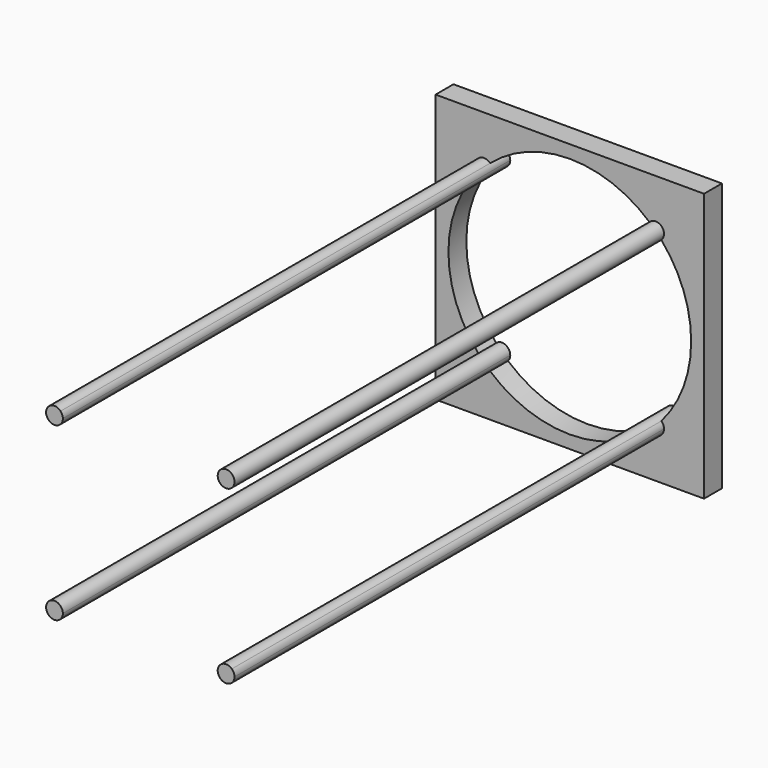
from build123d import *

# Parameters (mm, degrees)
F1_DEPTH = 635
F0_W     = 304.8
F0_H     = 304.8
F2_DEPTH = 25.4


with BuildPart() as f1:
    # F0 (on Front) → F1 (new body)
    with BuildSketch(Plane.XZ):
        with BuildLine():
            ThreePointArc((79.0087948248, 92.4711311021), (79.2375540094, 79.2375540094), (92.4711311021, 79.0087948248))
            ThreePointArc((92.4711311021, 79.0087948248), (85.9727461002, 85.9727461002), (79.0087948248, 92.4711311021))
        make_face()
        with BuildLine():
            ThreePointArc((79.0087948248, 92.4711311021), (85.9727461002, 85.9727461002), (92.4711311021, 79.0087948248))
            ThreePointArc((92.4711311021, 79.0087948248), (94.708384089, 82.1761352526), (95.4977461002, 85.9727461002))
            ThreePointArc((95.4977461002, 85.9727461002), (89.4651656842, 94.834384236), (79.0087948248, 92.4711311021))
        make_face()
    extrude(amount=F1_DEPTH)


with BuildPart() as f1b:
    # F0 (on Front) → F1, piece 2 (new body)
    with BuildSketch(Plane.XZ):
        with BuildLine():
            ThreePointArc((95.4977461002, -108.898811727), (94.708384089, -105.1022008793), (92.4711311021, -101.9348604515))
            ThreePointArc((92.4711311021, -101.9348604515), (85.9727461002, -108.898811727), (79.0087948248, -115.3971967289))
            ThreePointArc((79.0087948248, -115.3971967289), (89.4651656842, -117.7604498627), (95.4977461002, -108.898811727))
        make_face()
        with BuildLine():
            ThreePointArc((79.0087948248, -115.3971967289), (85.9727461002, -108.898811727), (92.4711311021, -101.9348604515))
            ThreePointArc((92.4711311021, -101.9348604515), (79.2375540094, -102.1636196362), (79.0087948248, -115.3971967289))
        make_face()
    extrude(amount=F1_DEPTH)


with BuildPart() as f1c:
    # F0 (on Front) → F1, piece 3 (new body)
    with BuildSketch(Plane.XZ):
        with BuildLine():
            ThreePointArc((-99.373811727, 85.9727461002), (-100.0371735912, 89.4651656842), (-101.9348604515, 92.4711311021))
            ThreePointArc((-101.9348604515, 92.4711311021), (-108.898811727, 85.9727461002), (-115.3971967289, 79.0087948248))
            ThreePointArc((-115.3971967289, 79.0087948248), (-105.1022008793, 77.2371081114), (-99.373811727, 85.9727461002))
        make_face()
        with BuildLine():
            ThreePointArc((-115.3971967289, 79.0087948248), (-108.898811727, 85.9727461002), (-101.9348604515, 92.4711311021))
            ThreePointArc((-101.9348604515, 92.4711311021), (-115.6340038178, 92.707938191), (-115.3971967289, 79.0087948248))
        make_face()
    extrude(amount=F1_DEPTH)


with BuildPart() as f1d:
    # F0 (on Front) → F1, piece 4 (new body)
    with BuildSketch(Plane.XZ):
        with BuildLine():
            ThreePointArc((-115.3971967289, -101.9348604515), (-115.6340038178, -115.6340038178), (-101.9348604515, -115.3971967289))
            ThreePointArc((-101.9348604515, -115.3971967289), (-108.898811727, -108.898811727), (-115.3971967289, -101.9348604515))
        make_face()
        with BuildLine():
            ThreePointArc((-115.3971967289, -101.9348604515), (-108.898811727, -108.898811727), (-101.9348604515, -115.3971967289))
            ThreePointArc((-101.9348604515, -115.3971967289), (-100.0371735912, -112.391231311), (-99.373811727, -108.898811727))
            ThreePointArc((-99.373811727, -108.898811727), (-105.1022008793, -100.1631737382), (-115.3971967289, -101.9348604515))
        make_face()
    extrude(amount=F1_DEPTH)


with BuildPart() as f2:
    # F0 (on Front) → F2 (new body)
    with BuildSketch(Plane.XZ):
        with Locations((-11.4630328134, -11.4630328134)):
            Rectangle(F0_W, F0_H)
        with BuildLine():
            ThreePointArc((92.4711311021, 79.0087948248), (117.5894180385, 36.8373497331), (126.3319671866, -11.4630328134))
            ThreePointArc((126.3319671866, -11.4630328134), (117.5894180385, -59.7634153598), (92.4711311021, -101.9348604515))
            ThreePointArc((92.4711311021, -101.9348604515), (94.708384089, -105.1022008793), (95.4977461002, -108.898811727))
            ThreePointArc((95.4977461002, -108.898811727), (89.4651656842, -117.7604498627), (79.0087948248, -115.3971967289))
            ThreePointArc((79.0087948248, -115.3971967289), (-11.4630328134, -149.2580328134), (-101.9348604515, -115.3971967289))
            ThreePointArc((-101.9348604515, -115.3971967289), (-115.6340038178, -115.6340038178), (-115.3971967289, -101.9348604515))
            ThreePointArc((-115.3971967289, -101.9348604515), (-149.2580328134, -11.4630328134), (-115.3971967289, 79.0087948248))
            ThreePointArc((-115.3971967289, 79.0087948248), (-115.6340038178, 92.707938191), (-101.9348604515, 92.4711311021))
            ThreePointArc((-101.9348604515, 92.4711311021), (-11.4630328134, 126.3319671866), (79.0087948248, 92.4711311021))
            ThreePointArc((79.0087948248, 92.4711311021), (89.4651656842, 94.834384236), (95.4977461002, 85.9727461002))
            ThreePointArc((95.4977461002, 85.9727461002), (94.708384089, 82.1761352526), (92.4711311021, 79.0087948248))
        make_face(mode=Mode.SUBTRACT)
    extrude(amount=F2_DEPTH)


solid = Compound([f1.part, f1b.part, f1c.part, f1d.part, f2.part])
